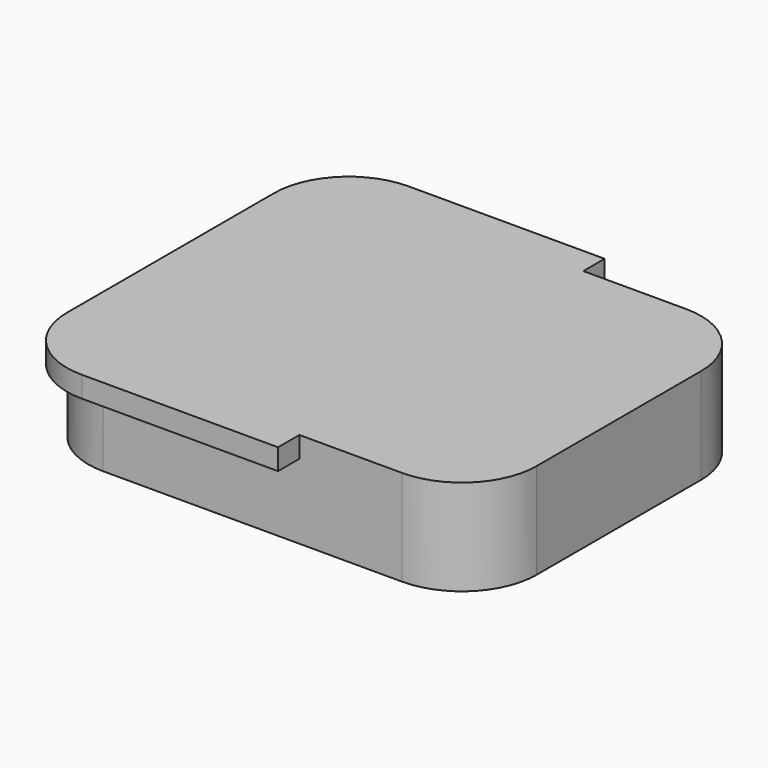
from build123d import *

# Parameters (mm, degrees)
F1_DEPTH     = 10.25
F3_DEPTH     = 2.25
F4_T         = 2.25
F4_T3_DEPTH  = 25.5
F4_T5_DEPTH  = 6.75
F4_T8_ANGLE  = 90.000000001
F4_T10_ANGLE = 90.000000001


# Not quite as in the source:
# - a shell that OpenCascade refuses in one call is made with other operations: the cavity is built on its own and cut out


with BuildPart() as f1:
    # F0 (on Top) → F1 (new body)
    with BuildSketch(Plane.XY):
        with BuildLine():
            Line((16, 19), (-16, 19))
            ThreePointArc((-16, 19), (-21.6568542495, 16.6568542495), (-24, 11))
            Line((-24, 11), (-24, -11))
            ThreePointArc((-24, -11), (-21.6568542495, -16.6568542495), (-16, -19))
            Line((-16, -19), (16, -19))
            ThreePointArc((16, -19), (21.6568542495, -16.6568542495), (24, -11))
            Line((24, -11), (24, 11))
            ThreePointArc((24, 11), (21.6568542495, 16.6568542495), (16, 19))
        make_face()
    extrude(amount=F1_DEPTH)

    # F2 (on face) → F3 (join)
    with BuildSketch(Plane.XY.offset(10.25)):
        with BuildLine():
            Line((5, 21.85), (-16, 21.85))
            ThreePointArc((-16, 21.85), (-21.6568542495, 19.5068542495), (-24, 13.85))
            Line((-24, 13.85), (-24, -13.85))
            ThreePointArc((-24, -13.85), (-21.6568542495, -19.5068542495), (-16, -21.85))
            Line((-16, -21.85), (5, -21.85))
            Line((5, -21.85), (5, 21.85))
        make_face()
    extrude(amount=-F3_DEPTH)

    # F4: shell of thickness 2.25, made by hand


with BuildPart() as f4_core1:
    # F4_t2: copy of F1
    add(f1.part)

    # the walls: a layer under each face that stays
    f4_faces = [f4_core1.faces().sort_by_distance(p)[0] for p in [
        (0, 19, 5.125),
        (21.6568542495, 16.6568542495, 5.125),
        (24, 0, 5.125),
        (21.6568542495, -16.6568542495, 5.125),
        (0, -19, 5.125),
        (-21.6568542495, -16.6568542495, 4),
        (-24, 0, 5.125),
        (-21.6568542495, -19.5068542495, 9.125),
        (-5.5, -21.85, 9.125),
        (-21.6568542495, 19.5068542495, 9.125),
        (-5.5, 21.85, 9.125),
        (-19.1666666667, -20.0416666667, 8),
        (5, -20.425, 9.125),
        (0, 0, 10.25),
        (5, 20.425, 9.125),
        (-19.1666666667, 20.0416666667, 8),
        (-21.6568542495, 16.6568542495, 4),
    ]]
    thicken(f4_faces, amount=-F4_T, mode=Mode.SUBTRACT)

    # F4_s4 → F4_t3 (cut)
    with BuildSketch(Plane.YZ.offset(-18.25)):
        Polygon((19.0225, 7.9775), (16.75, 8), (16.75, 10.25), (19, 10.25), align=None)
        Polygon((-19.0225, 7.9775), (-16.75, 8), (-16.75, 10.25), (-19, 10.25), align=None)
    extrude(amount=F4_T3_DEPTH, mode=Mode.SUBTRACT)

    # F4_s6 → F4_t5 (cut)
    with BuildSketch(Plane.XY.offset(5.75)):
        Polygon((5.0225, 19.0225), (5, 16.75), (2.75, 16.75), (2.75, 19), align=None)
        Polygon((5.0225, -19.0225), (5, -16.75), (2.75, -16.75), (2.75, -19), align=None)
    extrude(amount=F4_T5_DEPTH, mode=Mode.SUBTRACT)

    # F4_s7 → F4_t8 (revolve, cut)
    with BuildSketch(Plane.YZ.offset(-16)):
        Polygon((-19.0225, 7.9775), (-16.75, 8), (-16.75, 10.25), (-19, 10.25), align=None)
    revolve(axis=Axis((-16, -11, 8), (0, 0, -1)), revolution_arc=F4_T8_ANGLE, mode=Mode.SUBTRACT)

    # F4_s9 → F4_t10 (revolve, cut)
    with BuildSketch(Plane.XZ.offset(-11)):
        Polygon((-24.0225, 7.9775), (-24, 10.25), (-21.75, 10.25), (-21.75, 8), align=None)
    revolve(axis=Axis((-16, 11, 8), (0, 0, -1)), revolution_arc=F4_T10_ANGLE, mode=Mode.SUBTRACT)


with BuildPart() as f1_1:
    add(f1.part)

    # what is left inside the walls is the cavity
    f4_cavity = [f4_core1.part.solids().sort_by_distance(p)[0] for p in [
        (0, -5.583333, 7.9775),
    ]]
    add(f4_cavity, mode=Mode.SUBTRACT)


solid = f1_1.part
